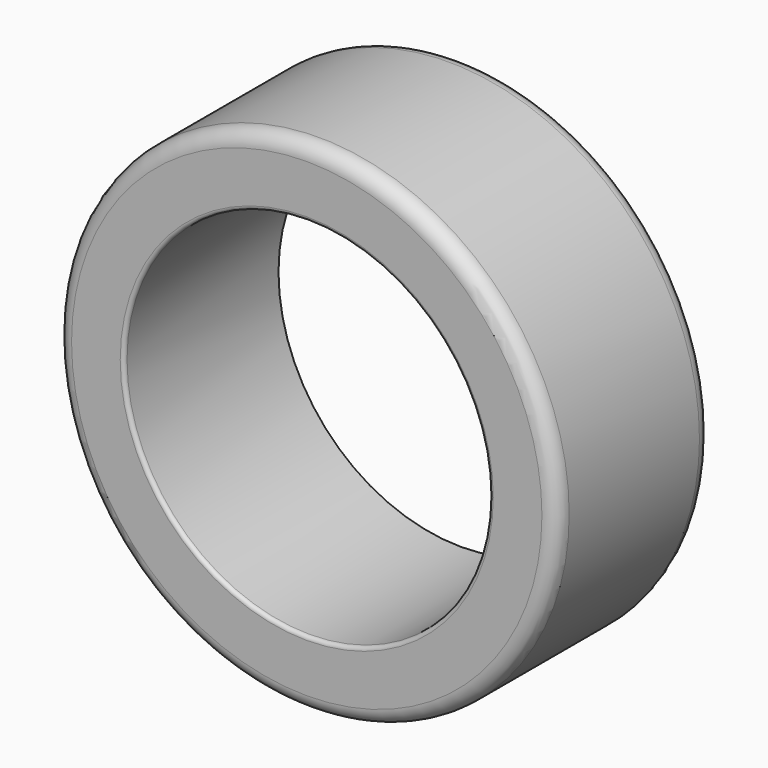
from build123d import *

# Parameters (mm, degrees)
F0_R     = 83.9597
F1_DEPTH = 32.385
F2_R     = 61.2902
F3_DEPTH = 50.8
F4_R     = 5.08
F5_R     = 1.27


with BuildPart() as f1:
    # F0 (on Front) → F1 (new body, symmetric)
    with BuildSketch(Plane.XZ):
        Circle(F0_R)
    extrude(amount=F1_DEPTH, both=True)

    # F2 (on Front) → F3 (cut, symmetric)
    with BuildSketch(Plane.XZ):
        Circle(F2_R)
    extrude(amount=F3_DEPTH, both=True, mode=Mode.SUBTRACT)

    # F4
    f4_edges = [f1.edges().sort_by_distance(p)[0] for p in [
        (-83.9597, -32.385, 0),
        (-83.9597, 32.385, 0),
    ]]
    fillet(f4_edges, radius=F4_R)

    # F5
    f5_edges = [f1.edges().sort_by_distance(p)[0] for p in [
        (-61.2902, -32.385, 0),
    ]]
    fillet(f5_edges, radius=F5_R)


solid = f1.part
